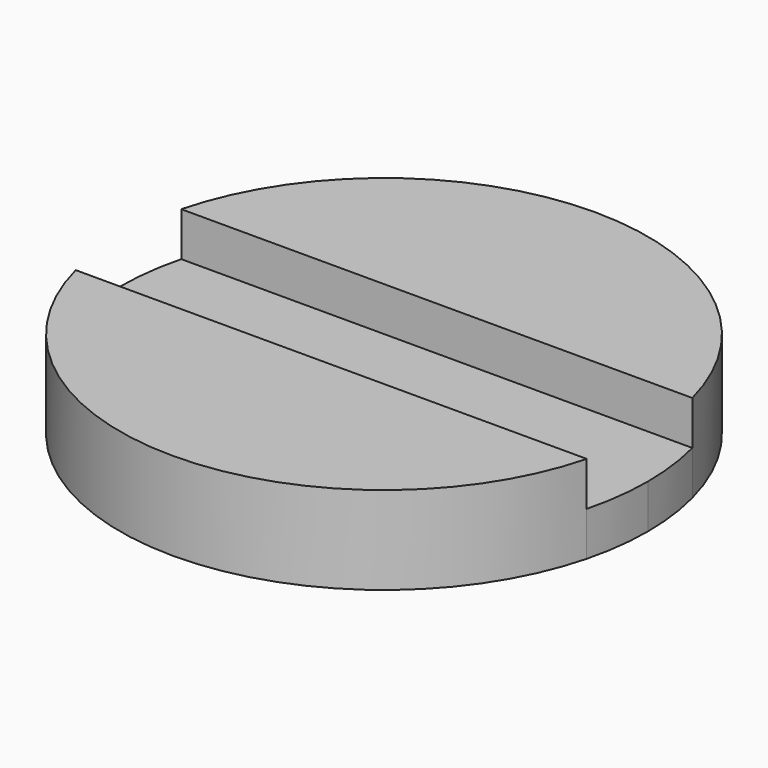
from build123d import *

# Parameters (mm, degrees)
F1_DEPTH = 3.175
F0_W     = 36.8901663726
F0_H     = 9.525
F2_DEPTH = 3.175


with BuildPart() as f1:
    # F0 (on Top) → F1 (new body)
    with BuildSketch(Plane.XY):
        with BuildLine():
            Line((-18.4450831863, 4.7625), (18.4450831863, 4.7625))
            ThreePointArc((18.4450831863, 4.7625), (0, 19.05), (-18.4450831863, 4.7625))
        make_face()
    extrude(amount=F1_DEPTH)



with BuildPart() as f1b:
    # F0 (on Top) → F1, piece 2 (new body)
    with BuildSketch(Plane.XY):
        with BuildLine():
            ThreePointArc((-18.4450831863, -4.7625), (0, -19.05), (18.4450831863, -4.7625))
            Line((18.4450831863, -4.7625), (-18.4450831863, -4.7625))
        make_face()
    extrude(amount=F1_DEPTH)


with BuildPart() as f1_1:
    add(f1.part)

    add(f1b.part)  # F2 merges F1b
    # F0 (on Top) → F2 (join)
    with BuildSketch(Plane.XY):
        with BuildLine():
            ThreePointArc((18.4450831863, -4.7625), (18.8981657139, -2.4003817718), (19.05, 0))
            ThreePointArc((19.05, 0), (18.8981657139, 2.4003817718), (18.4450831863, 4.7625))
            Line((18.4450831863, 4.7625), (18.4450831863, -4.7625))
        make_face()
        with BuildLine():
            Line((-18.4450831863, 4.7625), (18.4450831863, 4.7625))
            ThreePointArc((18.4450831863, 4.7625), (0, 19.05), (-18.4450831863, 4.7625))
        make_face()
        Rectangle(F0_W, F0_H)
        with BuildLine():
            ThreePointArc((-18.4450831863, -4.7625), (0, -19.05), (18.4450831863, -4.7625))
            Line((18.4450831863, -4.7625), (-18.4450831863, -4.7625))
        make_face()
        with BuildLine():
            Line((-18.4450831863, -4.7625), (-18.4450831863, 4.7625))
            ThreePointArc((-18.4450831863, 4.7625), (-19.05, 0), (-18.4450831863, -4.7625))
        make_face()
    extrude(amount=-F2_DEPTH)


solid = f1_1.part
